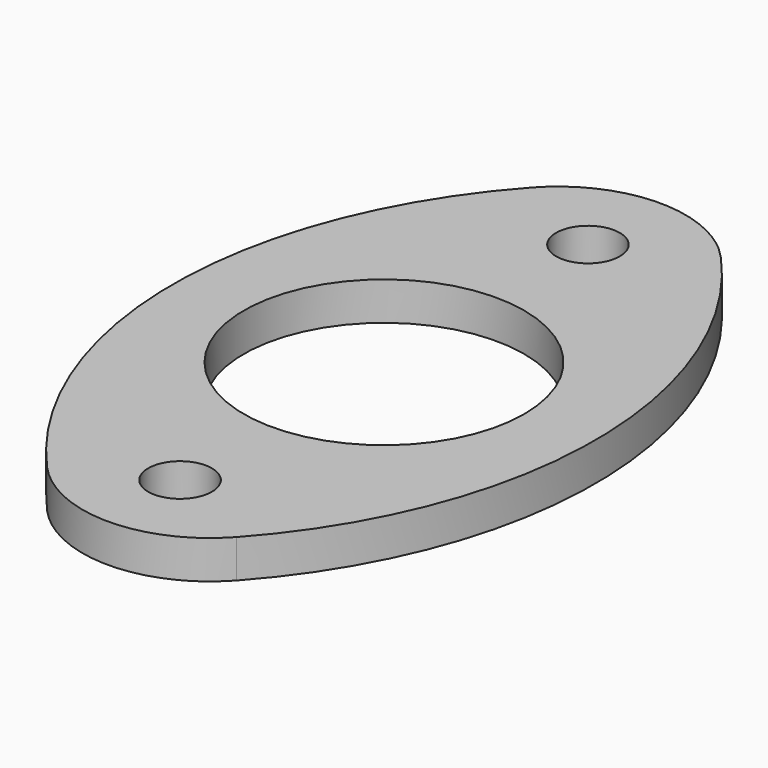
from build123d import *

# Parameters (mm, degrees)
F0_R     = 1.25
F0_R_2   = 5.5
F1_DEPTH = 1.5
F2_R     = 5


with BuildPart() as f1:
    # F0 (on Top) → F1 (new body)
    with BuildSketch(Plane.XY):
        with BuildLine():
            ThreePointArc((0, -15), (8.2826006835, 0), (0, 15))
            ThreePointArc((0, 15), (-8.2826006835, 0), (0, -15))
        make_face()
        with Locations((0, -10)):
            Circle(F0_R, mode=Mode.SUBTRACT)
        Circle(F0_R_2, mode=Mode.SUBTRACT)
        with Locations((0, 10)):
            Circle(F0_R, mode=Mode.SUBTRACT)
    extrude(amount=F1_DEPTH)

    # F2
    f2_edges = [f1.edges().sort_by_distance(p)[0] for p in [
        (0, -15, 0.75),
        (0, 15, 0.75),
    ]]
    fillet(f2_edges, radius=F2_R)


solid = f1.part
